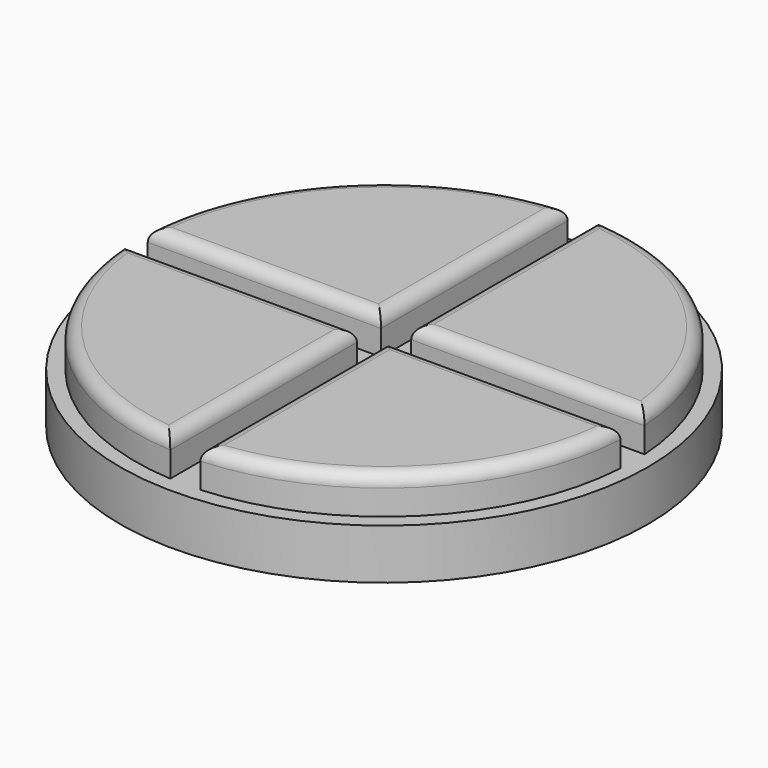
from build123d import *

# Parameters (mm, degrees)
F0_R     = 10.5
F1_DEPTH = 2
F3_DEPTH = 1.5
F4_R     = 0.5


with BuildPart() as f1:
    # F0 (on Top) → F1 (new body)
    with BuildSketch(Plane.XY):
        Circle(F0_R)
    extrude(amount=F1_DEPTH)

    # F2 (on face) → F3 (join)
    with BuildSketch(Plane.XY.offset(2)):
        with BuildLine():
            ThreePointArc((-9.8818014552, -0.6), (-7.0003571337, -7.0003571337), (-0.6, -9.8818014552))
            Line((-0.6, -9.8818014552), (-0.6, -0.6))
            Line((-0.6, -0.6), (-9.8818014552, -0.6))
        make_face()
        with BuildLine():
            Line((-0.6, 0.6), (-0.6, 9.8818014552))
            ThreePointArc((-0.6, 9.8818014552), (-7.0003571337, 7.0003571337), (-9.8818014552, 0.6))
            Line((-9.8818014552, 0.6), (-0.6, 0.6))
        make_face()
        with BuildLine():
            Line((0.6, 0.6), (9.8818014552, 0.6))
            ThreePointArc((9.8818014552, 0.6), (7.0003571337, 7.0003571337), (0.6, 9.8818014552))
            Line((0.6, 9.8818014552), (0.6, 0.6))
        make_face()
        with BuildLine():
            ThreePointArc((0.6, -9.8818014552), (7.0003571337, -7.0003571337), (9.8818014552, -0.6))
            Line((9.8818014552, -0.6), (0.6, -0.6))
            Line((0.6, -0.6), (0.6, -9.8818014552))
        make_face()
    extrude(amount=F3_DEPTH)

    # F4
    f4_edges = [f1.edges().sort_by_distance(p)[0] for p in [
        (-7.000357, -7.000357, 3.5),
        (-0.6, -5.240901, 3.5),
        (-5.240901, -0.6, 3.5),
        (-5.240901, 0.6, 3.5),
        (-0.6, 5.240901, 3.5),
        (5.240901, 0.6, 3.5),
        (0.6, 5.240901, 3.5),
        (5.240901, -0.6, 3.5),
        (0.6, -5.240901, 3.5),
        (7.000357, 7.000357, 3.5),
        (7.000357, -7.000357, 3.5),
        (-7.000357, 7.000357, 3.5),
    ]]
    fillet(f4_edges, radius=F4_R)


solid = f1.part
